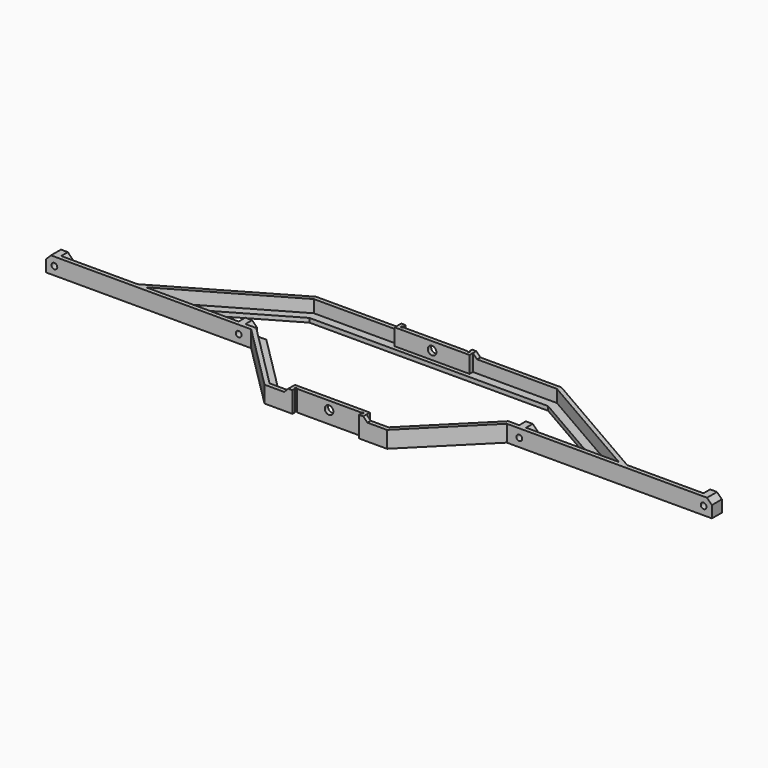
from build123d import *

# Parameters (mm, degrees)
F1_DEPTH  = 1.5875
F3_DEPTH  = 4.7625
F4_W      = 6.35
F4_H      = 6.35
F5_DEPTH  = 3.175
F6_SIZE   = 1.8598642
F7_W      = 28.575
F7_H      = 3.175
F8_DEPTH  = 1.5875
F9_W      = 25.4
F9_H      = 1.5875
F10_DEPTH = 7.9375
F11_R     = 1.0922
F11_R_2   = 1.63322
F12_DEPTH = 28.575
F13_SIZE  = 1.58749
F14_R     = 0.396875
F15_DEPTH = 7.9375
F16_R     = 1.63322
F17_DEPTH = 1.5875


# Not quite as in the source:
# - a fillet or chamfer is up to 0.001 mm smaller than in the source, because OpenCascade refuses the exact size


with BuildPart() as f1:
    # F0 (on Top) → F1 (new body)
    with BuildSketch(Plane.XY):
        Polygon((-87.87765, 25.4), (-127, 25.4), (-127, 20.6375), (-48.7553, 20.6375), (-23.3553, -4.7625), (23.3553, -4.7625), (48.7553, 20.6375), (127, 20.6375), (127, 25.4), (87.87765, 25.4), (46.7826079092, 49.1262336135), (-46.7826079092, 49.1262336135), align=None)
        Polygon((-21.3826079092, 0), (-46.7826079092, 25.4), (-78.35265, 25.4), (-45.5064998802, 44.3637336135), (45.5064998802, 44.3637336135), (78.35265, 25.4), (46.7826079092, 25.4), (21.3826079092, 0), align=None, mode=Mode.SUBTRACT)
    extrude(amount=F1_DEPTH)

    # F2 (on face) → F3 (join)
    with BuildSketch(Plane.XY.offset(1.5875)):
        Polygon((-127, 22.225), (-127, 20.6375), (-48.7553, 20.6375), (-23.3553, -4.7625), (23.3553, -4.7625), (48.7553, 20.6375), (127, 20.6375), (127, 22.225), (93.376911314, 22.225), (87.87765, 25.4), (46.7826079092, 49.1262336135), (-46.7826079092, 49.1262336135), (-87.87765, 25.4), (-93.376911314, 22.225), align=None)
        Polygon((90.201911314, 22.225), (48.0977359697, 22.225), (22.6977359697, -3.175), (14.2875, -3.175), (14.2875, -1.5875), (-14.2875, -1.5875), (-14.2875, -3.175), (-22.6977359697, -3.175), (-48.0977359697, 22.225), (-90.201911314, 22.225), (-46.3572385662, 47.5387336135), (-14.2875, 47.5387336135), (-14.2875, 45.9512336135), (14.2875, 45.9512336135), (14.2875, 47.5387336135), (46.3572385662, 47.5387336135), align=None, mode=Mode.SUBTRACT)
    extrude(amount=F3_DEPTH)

    # F4 (on face) → F5 (join, through all)
    with BuildSketch(Plane(origin=(0, 22.225, 0), x_dir=(-1, 0, 0), z_dir=(0, 1, 0))):
        with Locations((-53.5178, 3.175)):
            Rectangle(F4_W, F4_H)
        with Locations((-123.825, 3.175)):
            Rectangle(F4_W, F4_H)
        with Locations((123.825, 3.175)):
            Rectangle(F4_W, F4_H)
        with Locations((53.5178, 3.175)):
            Rectangle(F4_W, F4_H)
    extrude(amount=F5_DEPTH)

    # F6
    f6_edges = [f1.edges().sort_by_distance(p)[0] for p in [
        (-127, 23.01875, 6.35),
        (-120.65, 23.8125, 6.35),
        (-56.6928, 23.8125, 6.35),
        (-50.3428, 23.8125, 6.35),
        (50.3428, 23.8125, 6.35),
        (56.6928, 23.8125, 6.35),
        (120.65, 23.8125, 6.35),
        (127, 23.01875, 6.35),
    ]]
    chamfer(f6_edges, length=F6_SIZE)

    # F7 (on face) → F8 (join)
    with BuildSketch(Plane.XY.offset(6.35)):
        with Locations((0, -3.175)):
            Rectangle(F7_W, F7_H)
        with Locations((0, 47.5387336135)):
            Rectangle(F7_W, F7_H)
    extrude(amount=F8_DEPTH)

    # F9 (on face) → F10 (cut, through all)
    with BuildSketch(Plane.XY.offset(7.9375)):
        with Locations((0, -3.96875)):
            Rectangle(F9_W, F9_H)
        with Locations((0, 48.3324836135)):
            Rectangle(F9_W, F9_H)
    extrude(amount=-F10_DEPTH, mode=Mode.SUBTRACT)

    # F11 (on face) → F12 (cut, through all)
    with BuildSketch(Plane.XZ.offset(3.175)):
        with Locations((53.5178, 3.175)):
            Circle(F11_R)
        with Locations((123.825, 3.175)):
            Circle(F11_R)
        with Locations((-123.825, 3.175)):
            Circle(F11_R)
        with Locations((-53.5178, 3.175)):
            Circle(F11_R)
        with Locations((0, 4.7625)):
            Circle(F11_R_2)
    extrude(amount=-F12_DEPTH, mode=Mode.SUBTRACT)

    # F13 (size 1.5875 in the source; OpenCascade refuses exactly that, so slightly less here)
    f13_edges = [f1.edges().sort_by_distance(p)[0] for p in [
        (-14.2875, -3.96875, 6.35),
        (14.2875, -3.96875, 6.35),
        (-14.2875, 48.332484, 6.35),
        (14.2875, 48.332484, 6.35),
    ]]
    chamfer(f13_edges, length=F13_SIZE)

    # F14 (on face) → F15 (cut, through all)
    with BuildSketch(Plane.XY.offset(7.9375)):
        with Locations((-12.7, -3.175)):
            Circle(F14_R)
        with Locations((12.7, -3.175)):
            Circle(F14_R)
        with Locations((12.7, 47.5387336135)):
            Circle(F14_R)
        with Locations((-12.7, 47.5387336135)):
            Circle(F14_R)
    extrude(amount=-F15_DEPTH, mode=Mode.SUBTRACT)

    # F16 (on face) → F17 (cut, through all)
    with BuildSketch(Plane(origin=(0, 47.5387336135, 0), x_dir=(-1, 0, 0), z_dir=(0, 1, 0))):
        with Locations((0, 4.7625)):
            Circle(F16_R)
    extrude(amount=-F17_DEPTH, mode=Mode.SUBTRACT)


solid = f1.part
